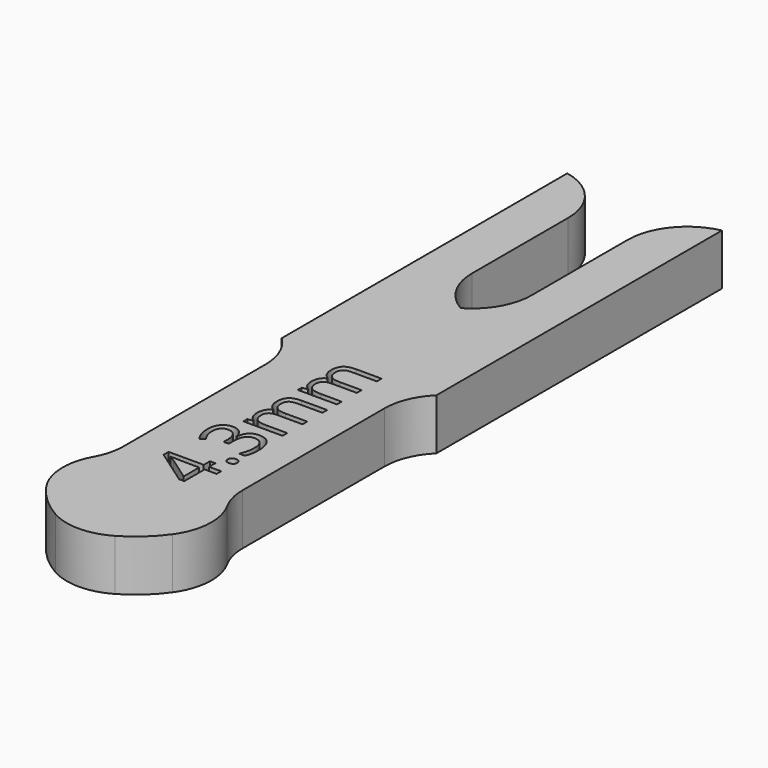
from build123d import *

# Parameters (mm, degrees)
F1_DEPTH     = 4.3
F2_TEXT_SIZE = 6.1470489363
F3_DEPTH     = 1
F4_T1_DEPTH  = 49.3
F4_T3_DEPTH  = 32.5842712475
F5_R         = 5
F6_T1_DEPTH  = 4.3
F7_T1_DEPTH  = 28.7948974279
F8_T1_DEPTH  = 4.3


# Not quite as in the source:
# - a fillet or chamfer that OpenCascade refuses, or shapes differently, is made with other operations: its cross-section is extruded or revolved along the edge and cut away or added
# - Text() gives the source's letters only with a copy of the font that has no kerning and outlines rounded to 1/6400 em; it was checked with that copy


with BuildPart() as f1:
    # F0 (on Top) → F1 (new body)
    with BuildSketch(Plane.XY):
        Polygon((-7, 0), (0, 0), (7, 0), (7, 10), (5, 10), (5, 30), (6.5, 30), (6.5, 60), (2.5, 60), (2.5, 40), (0, 40), (-2.5, 40), (-2.5, 60), (-6.5, 60), (-6.5, 30), (-5, 30), (-5, 10), (-7, 10), align=None)
    extrude(amount=F1_DEPTH)

    # F2 (on face) → F3 (cut)
    with BuildSketch(Plane.XY.offset(4.3)):
        with Locations(Location((2.2129376171, 10), (0, 0, 90))):
            Text('4.3mm', F2_TEXT_SIZE, font='Open Sans', text_align=(TextAlign.LEFT, TextAlign.BOTTOM))
    extrude(amount=-F3_DEPTH, mode=Mode.SUBTRACT)

    # F4: fillet of radius 9 on 4 edges, made by hand

    # F4_s2 → F4_t1 (cut)
    with BuildSketch(Plane.XY.offset(-22.5)):
        with BuildLine():
            ThreePointArc((-2, 0), (4.3639610307, 2.6360389693), (7, 9))
            Line((7, 9), (7, 0))
            Line((7, 0), (-2, 0))
        make_face()
        with BuildLine():
            ThreePointArc((2, 0), (-4.3639610307, 2.6360389693), (-7, 9))
            Line((-7, 9), (-7, 0))
            Line((-7, 0), (2, 0))
        make_face()
    extrude(amount=F4_T1_DEPTH, mode=Mode.SUBTRACT)

    # F4_s4 → F4_t3 (cut)
    with BuildSketch(Plane.XY.offset(-14.1421356237)):
        with BuildLine():
            ThreePointArc((7, 4.3431457505), (6.4852813742, 7.3431457505), (5, 10))
            Line((5, 10), (7, 10))
            Line((7, 10), (7, 4.3431457505))
        make_face()
        with BuildLine():
            ThreePointArc((-7, 4.3431457505), (-6.4852813742, 7.3431457505), (-5, 10))
            Line((-5, 10), (-7, 10))
            Line((-7, 10), (-7, 4.3431457505))
        make_face()
    extrude(amount=F4_T3_DEPTH, mode=Mode.SUBTRACT)

    # F5
    f5_edges = [f1.edges().sort_by_distance(p)[0] for p in [
        (0, 0.225036, 2.15),
        (6.693585, 6.671573, 2.15),
        (-6.693585, 6.671573, 2.15),
    ]]
    fillet(f5_edges, radius=F5_R)

    # F6: fillet of radius 5 on 4 edges, made by hand

    # F6_s2 → F6_t1 (join)
    with BuildSketch(Plane.XY):
        with BuildLine():
            ThreePointArc((5.6262247019, 9.0943996627), (5.1590870443, 10.2660023476), (5, 11.5172264502))
            Line((5, 11.5172264502), (4.5, 11.5172264502))
            Line((4.5, 11.5172264502), (4.5, 10))
            Line((4.5, 10), (4.6111111111, 9.6857303195))
            ThreePointArc((4.6111111111, 9.6857303195), (4.9114549834, 9.2910533904), (5.1888471721, 8.8521169839))
            Line((5.1888471721, 8.8521169839), (5.6262247019, 9.0943996627))
        make_face()
        with BuildLine():
            ThreePointArc((-5.6262247019, 9.0943996627), (-5.1590870443, 10.2660023476), (-5, 11.5172264502))
            Line((-5, 11.5172264502), (-4.5, 11.5172264502))
            Line((-4.5, 11.5172264502), (-4.5, 10))
            Line((-4.5, 10), (-4.6111111111, 9.6857303195))
            ThreePointArc((-4.6111111111, 9.6857303195), (-4.9114549834, 9.2910533904), (-5.1888471721, 8.8521169839))
            Line((-5.1888471721, 8.8521169839), (-5.6262247019, 9.0943996627))
        make_face()
        with BuildLine():
            ThreePointArc((-5, 26.4292857857), (-5.3902277714, 28.3657774588), (-6.5, 30))
            Line((-6.5, 30), (-5, 30))
            Line((-5, 30), (-5, 26.4292857857))
        make_face()
        with BuildLine():
            ThreePointArc((5, 26.4292857857), (5.3902277714, 28.3657774588), (6.5, 30))
            Line((6.5, 30), (5, 30))
            Line((5, 30), (5, 26.4292857857))
        make_face()
    extrude(amount=F6_T1_DEPTH)

    # F7: fillet of radius 5 on 2 edges, made by hand

    # F7_s2 → F7_t1 (cut)
    with BuildSketch(Plane.XY.offset(-12.2474487139)):
        with BuildLine():
            ThreePointArc((-6.5, 60), (-3.6270166538, 58.2632981746), (-2.5, 55.1010205144))
            Line((-2.5, 55.1010205144), (-2.5, 60))
            Line((-2.5, 60), (-6.5, 60))
        make_face()
        with BuildLine():
            ThreePointArc((2.5, 55.1010205144), (3.6270166538, 58.2632981746), (6.5, 60))
            Line((6.5, 60), (2.5, 60))
            Line((2.5, 60), (2.5, 55.1010205144))
        make_face()
    extrude(amount=F7_T1_DEPTH, mode=Mode.SUBTRACT)

    # F8: fillet of radius 5 on 2 edges, made by hand

    # F8_s2 → F8_t1 (join)
    with BuildSketch(Plane.XY):
        with BuildLine():
            ThreePointArc((-2.5, 45), (-1.0355339059, 41.4644660941), (2.5, 40))
            Line((2.5, 40), (-2.5, 40))
            Line((-2.5, 40), (-2.5, 45))
        make_face()
        with BuildLine():
            ThreePointArc((-2.5, 40), (1.0355339059, 41.4644660941), (2.5, 45))
            Line((2.5, 45), (2.5, 40))
            Line((2.5, 40), (-2.5, 40))
        make_face()
    extrude(amount=F8_T1_DEPTH)


solid = f1.part
